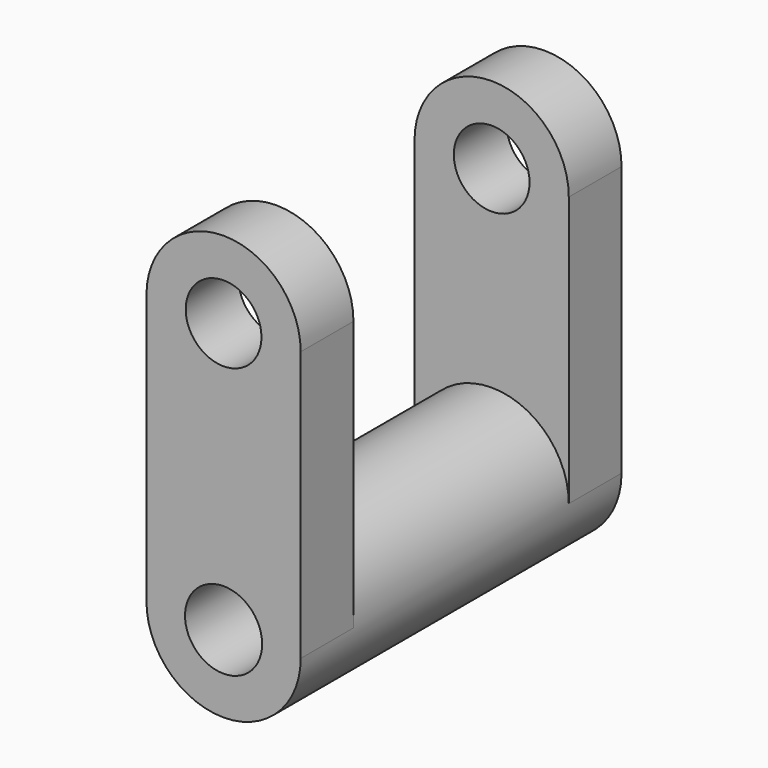
from build123d import *

# Parameters (mm, degrees)
F1_DEPTH = 17.1
F2_R     = 9.8201820523
F3_DEPTH = 25
F5_DEPTH = 34.9
F6_R     = 10
F7_DEPTH = 52.001


with BuildPart() as f1:
    # F0 (on Front) → F1 (new body)
    with BuildSketch(Plane.XZ):
        with BuildLine():
            Line((-18.8324629198, 51.7522737756), (-18.8324629198, -18.2477262244))
            ThreePointArc((-18.8324629198, -18.2477262244), (1.1675370802, -38.2477262244), (21.1675370802, -18.2477262244))
            Line((21.1675370802, -18.2477262244), (21.1675370802, 51.7522737756))
            ThreePointArc((21.1675370802, 51.7522737756), (1.1675370802, 71.7522737756), (-18.8324629198, 51.7522737756))
        make_face()
    extrude(amount=F1_DEPTH)

    # F2 (on face) → F3 (cut)
    with BuildSketch(Plane.XZ.offset(17.1)):
        with Locations((1.1675370802, 51.7522737756)):
            Circle(F2_R)
    extrude(amount=-F3_DEPTH, mode=Mode.SUBTRACT)

    # F4 (on face) → F5 (join)
    with BuildSketch(Plane(origin=(0, 0, 0), x_dir=(-1, 0, 0), z_dir=(0, 1, 0))):
        with BuildLine():
            ThreePointArc((-21.1675370802, -18.2477262244), (-1.1675370802, -38.2477262244), (18.8324629198, -18.2477262244))
            ThreePointArc((18.8324629198, -18.2477262244), (-1.1675370802, 1.7522737756), (-21.1675370802, -18.2477262244))
        make_face()
    extrude(amount=F5_DEPTH)

    # F6 (on face) → F7 (cut, through all)
    with BuildSketch(Plane.XZ.offset(17.1)):
        with Locations((1.1675370802, -18.2477262244)):
            Circle(F6_R)
    extrude(amount=-F7_DEPTH, mode=Mode.SUBTRACT)

    # F8: F1 across face


with BuildPart() as f1_1:
    add(f1.part)
    add(f1.part.mirror(Plane(origin=(1.1675370802, 34.9, -18.2477262244), x_dir=(-1, 0, 0), z_dir=(0, 1, 0))))


solid = f1_1.part
